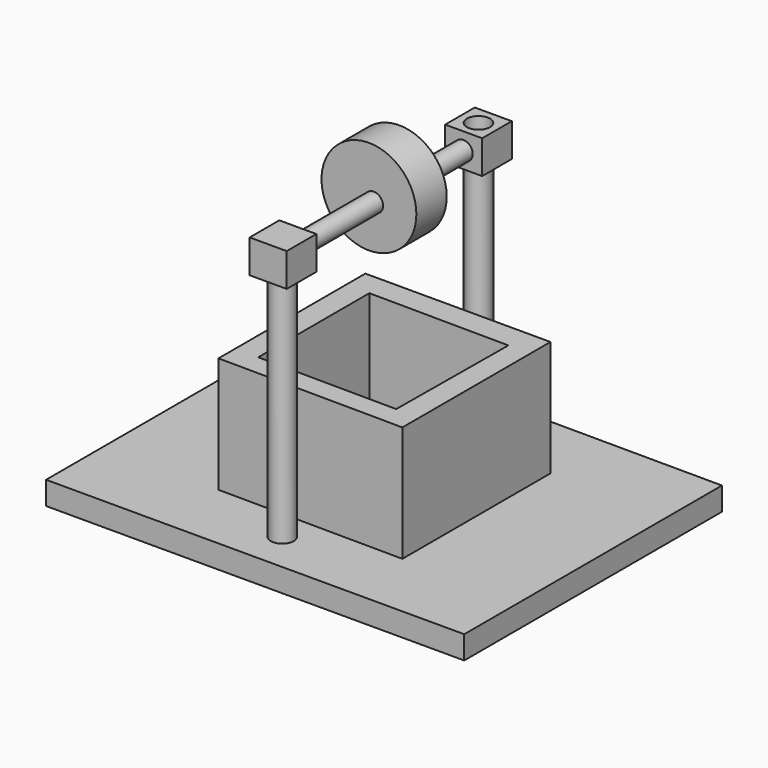
from build123d import *

# Parameters (mm, degrees)
F1_DEPTH  = 38.1
F3_DEPTH  = 6.35
F5_DEPTH  = 111.76
F6_R      = 3.175
F7_DEPTH  = 63.5
F8_R      = 3.175
F9_DEPTH  = 9.144
F10_R     = 2.5761417158
F11_DEPTH = 56.7944
F12_R     = 13.0117300102
F13_DEPTH = 33.274
F14_DEPTH = 22.86


with BuildPart() as f1:
    # F0 (on Top) → F1 (new body)
    with BuildSketch(Plane.XY):
        Polygon((-17.1450002551, 50.390333843), (-42.5450002551, 50.390333843), (-67.943348394, 50.390333843), (-67.943348394, 0), (-17.1450002551, -0.409666157), align=None)
    extrude(amount=F1_DEPTH)

    # F4 (on face) → F5 (cut)
    with BuildSketch(Plane.XY.offset(38.1)):
        Polygon((-61.593348394, 43.8162393793), (-61.593348394, 5.7150004432), (-23.4945872898, 5.4077508254), (-23.1873376721, 43.5065119296), align=None)
    extrude(amount=-F5_DEPTH, mode=Mode.SUBTRACT)


with BuildPart() as f3:
    # F2 (on Top) → F3 (new body)
    with BuildSketch(Plane.XY):
        Polygon((15.0603158399, 68.9530000091), (-99.6942445636, 69.448672235), (-99.6942445636, -19.439002499), (15.0603158399, -19.439002499), align=None)
    extrude(amount=F3_DEPTH)

    # F6 (on face) → F7 (join)
    with BuildSketch(Plane.XY.offset(6.35)):
        with Locations((-43.6241216958, 58.8009990752)):
            Circle(F6_R)
        with Locations((-43.6241216958, -8.508999832)):
            Circle(F6_R)
    extrude(amount=F7_DEPTH)

    # F8 (on face) → F9, piece 2 (join)
    with BuildSketch(Plane.XY.offset(69.85)):
        Polygon((-48.7041212618, -3.1750001945), (-48.7041212618, -7.4930000119), (-48.7041212618, -13.3350007236), (-38.5441212618, -13.3350007236), (-38.5441212618, -3.1750001945), align=None)
    extrude(amount=F9_DEPTH)

    # F10 (on face) → F11 (join)
    with BuildSketch(Plane(origin=(0, -3.1750001945, 0), x_dir=(-1, 0, 0), z_dir=(0, 1, 0))):
        with Locations((43.6241212618, 74.422)):
            Circle(F10_R)
    extrude(amount=F11_DEPTH)

    # F12 (on Front) → F13 (join)
    with BuildSketch(Plane.XZ):
        with Locations((-44.9327416718, 75.3640756011)):
            Circle(F12_R)
    extrude(amount=-F13_DEPTH)

    # F14 (cut): a face of the model
    f14_faces = [f3.faces().sort_by_distance(p)[0] for p in [
        (-57.576444381, 0, 75.3640756011),
    ]]
    extrude(f14_faces, amount=-F14_DEPTH, mode=Mode.SUBTRACT)


with BuildPart() as f9:
    # F8 (on face) → F9 (new body)
    with BuildSketch(Plane.XY.offset(69.85)):
        Polygon((-48.7041212618, 63.8810023665), (-48.7041212618, 59.8170012236), (-48.7041212618, 53.7210023665), (-38.5441212618, 53.7210023665), (-38.5441212618, 63.8810023665), align=None)
        with Locations((-43.6241216958, 58.8009990752)):
            Circle(F8_R, mode=Mode.SUBTRACT)
    extrude(amount=F9_DEPTH)


solid = Compound([f1.part, f3.part, f9.part])
